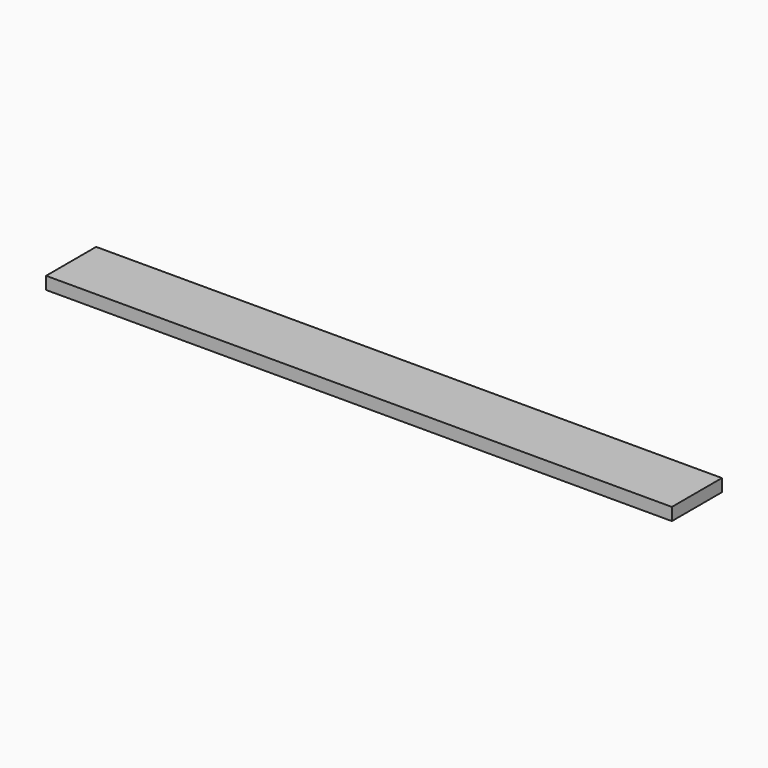
from build123d import *

# Parameters (mm, degrees)
F0_W     = 127
F0_H     = 12.7
F1_DEPTH = 2.54


# Not quite as in the source:
# - a feature names something its author has since deleted; it is built from what else it names


with BuildPart() as f1:
    # F0 (on Top) → F1 (new body)
    with BuildSketch(Plane.XY):
        with Locations((63.5, 6.35)):
            Rectangle(F0_W, F0_H)
    extrude(amount=F1_DEPTH)


solid = f1.part
